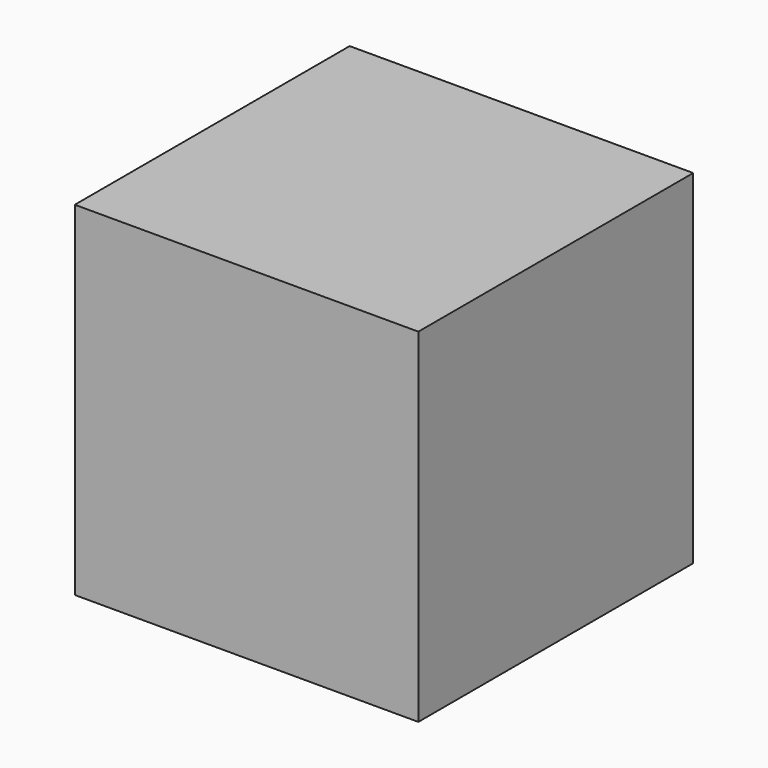
from build123d import *

# Parameters (mm, degrees)
F0_W     = 100
F0_H     = 100
F1_DEPTH = 50


# Not quite as in the source:
# - the program builds the solid bodies; features that only make, move or delete a surface that nothing else refers to are left out


with BuildPart() as f1:
    # F0 (on Top) → F1 (new body, symmetric)
    with BuildSketch(Plane.XY):
        Rectangle(F0_W, F0_H)
    extrude(amount=F1_DEPTH, both=True)


solid = f1.part
